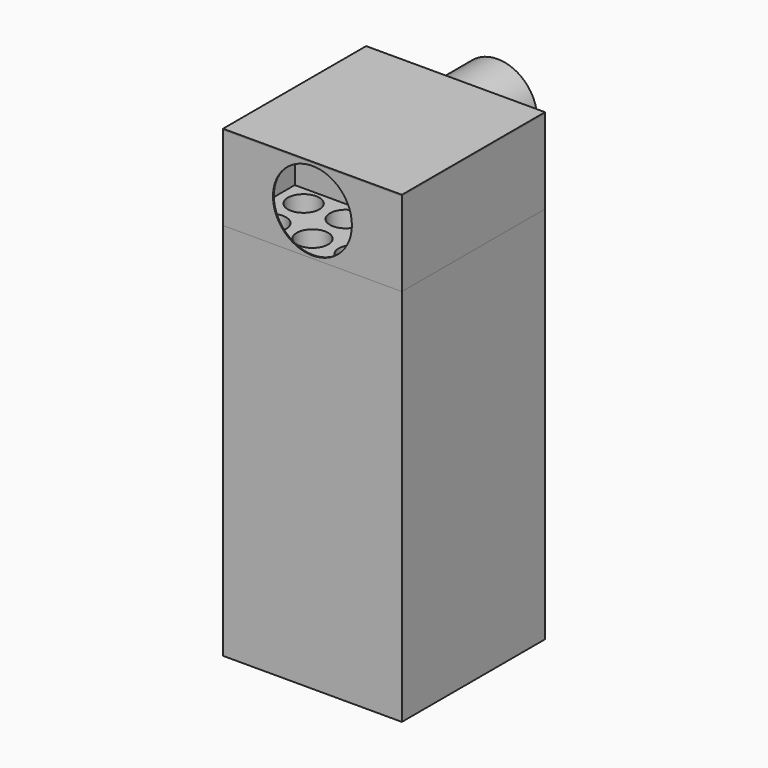
from build123d import *

# Parameters (mm, degrees)
F0_W           = 340
F0_H           = 340
F0_R           = 30
F1_DEPTH       = 360
F2_W           = 340
F2_H           = 340
F2_W_2         = 335.99999547
F2_H_2         = 335.99999547
F3_DEPTH       = 160
F4_W           = 2
F4_H           = 160
F5_DEPTH       = 336
F6_W           = 340
F6_H           = 340
F7_DEPTH       = 2
F8_R           = 75
F9_DEPTH       = 12.5
F12_R          = 75
F13_DEPTH      = 25
F14_R          = 75
F14_R_2        = 71.9999969006
F15_DEPTH      = 100
F15_DEPTH_BACK = 4
F16_W          = 336
F16_H          = 336
F16_R          = 31.4999952912
F17_DEPTH      = 718


# Not quite as in the source:
# - the program builds the solid bodies; features that only make, move or delete a surface that nothing else refers to are left out


with BuildPart() as f1:
    # F0 (on Top) → F1 (new body, symmetric)
    with BuildSketch(Plane.XY):
        with Locations((0, -139.3003371358)):
            Rectangle(F0_W, F0_H)
        with Locations((-120, -259.3003371358)):
            Circle(F0_R, mode=Mode.SUBTRACT)
        with Locations((-40, -259.3003371358)):
            Circle(F0_R, mode=Mode.SUBTRACT)
        with Locations((-120.7945212722, -179.3003371358)):
            Circle(F0_R, mode=Mode.SUBTRACT)
        with Locations((-40.7945212722, -179.3003371358)):
            Circle(F0_R, mode=Mode.SUBTRACT)
        with Locations((40, -259.3003371358)):
            Circle(F0_R, mode=Mode.SUBTRACT)
        with Locations((120, -259.3003371358)):
            Circle(F0_R, mode=Mode.SUBTRACT)
        with Locations((39.2054787278, -179.3003371358)):
            Circle(F0_R, mode=Mode.SUBTRACT)
        with Locations((119.2054787278, -179.3003371358)):
            Circle(F0_R, mode=Mode.SUBTRACT)
        with Locations((-120, -99.3003371358)):
            Circle(F0_R, mode=Mode.SUBTRACT)
        with Locations((-40, -99.3003371358)):
            Circle(F0_R, mode=Mode.SUBTRACT)
        with Locations((-120, -19.3003371358)):
            Circle(F0_R, mode=Mode.SUBTRACT)
        with Locations((-40, -19.3003371358)):
            Circle(F0_R, mode=Mode.SUBTRACT)
        with Locations((40, -99.3003371358)):
            Circle(F0_R, mode=Mode.SUBTRACT)
        with Locations((120, -99.3003371358)):
            Circle(F0_R, mode=Mode.SUBTRACT)
        with Locations((40, -19.3003371358)):
            Circle(F0_R, mode=Mode.SUBTRACT)
        with Locations((120, -19.3003371358)):
            Circle(F0_R, mode=Mode.SUBTRACT)
    extrude(amount=F1_DEPTH, both=True)

    # F16 (on face) → F17 (cut)
    with BuildSketch(Plane(origin=(0, 0, -360), x_dir=(1, 0, 0), z_dir=(0, 0, -1))):
        with Locations((0, 139.3003371358)):
            Rectangle(F16_W, F16_H)
        with Locations((-120, 19.3003371358)):
            Circle(F16_R, mode=Mode.SUBTRACT)
        with Locations((-40, 19.3003371358)):
            Circle(F16_R, mode=Mode.SUBTRACT)
        with Locations((-120, 99.3003371358)):
            Circle(F16_R, mode=Mode.SUBTRACT)
        with Locations((-40, 99.3003371358)):
            Circle(F16_R, mode=Mode.SUBTRACT)
        with Locations((40, 19.3003371358)):
            Circle(F16_R, mode=Mode.SUBTRACT)
        with Locations((120, 19.3003371358)):
            Circle(F16_R, mode=Mode.SUBTRACT)
        with Locations((40, 99.3003371358)):
            Circle(F16_R, mode=Mode.SUBTRACT)
        with Locations((120, 99.3003371358)):
            Circle(F16_R, mode=Mode.SUBTRACT)
        with Locations((-120.7945212722, 179.3003371358)):
            Circle(F16_R, mode=Mode.SUBTRACT)
        with Locations((-40.7945212722, 179.3003371358)):
            Circle(F16_R, mode=Mode.SUBTRACT)
        with Locations((-120, 259.3003371358)):
            Circle(F16_R, mode=Mode.SUBTRACT)
        with Locations((-40, 259.3003371358)):
            Circle(F16_R, mode=Mode.SUBTRACT)
        with Locations((39.2054787278, 179.3003371358)):
            Circle(F16_R, mode=Mode.SUBTRACT)
        with Locations((119.2054787278, 179.3003371358)):
            Circle(F16_R, mode=Mode.SUBTRACT)
        with Locations((40, 259.3003371358)):
            Circle(F16_R, mode=Mode.SUBTRACT)
        with Locations((120, 259.3003371358)):
            Circle(F16_R, mode=Mode.SUBTRACT)
    extrude(amount=-F17_DEPTH, mode=Mode.SUBTRACT)


with BuildPart() as f3:
    # F2 (on face) → F3 (new body)
    with BuildSketch(Plane.XY.offset(360)):
        with Locations((0, -139.3003371358)):
            Rectangle(F2_W, F2_H)
        with Locations((0, -139.3003371358)):
            Rectangle(F2_W_2, F2_H_2, mode=Mode.SUBTRACT)
    extrude(amount=F3_DEPTH)

    # F8 (on face) → F9 (cut, symmetric)
    with BuildSketch(Plane.XZ.offset(309.3003371358)):
        with Locations((0, 440)):
            Circle(F8_R)
    extrude(amount=F9_DEPTH, both=True, mode=Mode.SUBTRACT)

    # F12 (on face) → F13 (cut)
    with BuildSketch(Plane(origin=(0, 30.6996628642, 0), x_dir=(-1, 0, 0), z_dir=(0, 1, 0))):
        with Locations((0, 440)):
            Circle(F12_R)
    extrude(amount=-F13_DEPTH, mode=Mode.SUBTRACT)

    # F14 (on face) → F15 (join, two sides)
    with BuildSketch(Plane(origin=(0, 30.6996628642, 0), x_dir=(-1, 0, 0), z_dir=(0, 1, 0))) as f15_sk:
        with Locations((0, 440)):
            Circle(F14_R)
        with Locations((0, 440)):
            Circle(F14_R_2, mode=Mode.SUBTRACT)
    extrude(amount=F15_DEPTH)
    extrude(f15_sk.sketch, amount=-F15_DEPTH_BACK)


with BuildPart() as f5:
    # F4 (on face) → F5 (new body)
    with BuildSketch(Plane(origin=(167.999997735, 0, 0), x_dir=(0, -1, 0), z_dir=(-1, 0, 0))):
        with Locations((140.3003371358, 440)):
            Rectangle(F4_W, F4_H)
    extrude(amount=F5_DEPTH)


with BuildPart() as f7:
    # F6 (on face) → F7 (new body)
    with BuildSketch(Plane.XY.offset(520)):
        with Locations((0, -139.3003371358)):
            Rectangle(F6_W, F6_H)
    extrude(amount=F7_DEPTH)


solid = Compound([f1.part, f3.part, f5.part, f7.part])
